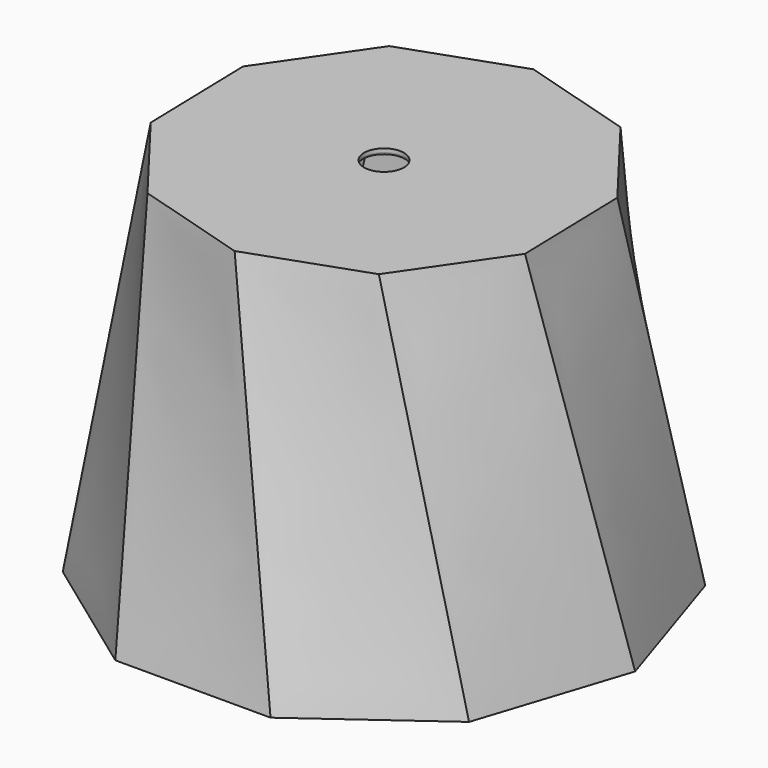
from build123d import *

# Parameters (mm, degrees)
F4_T     = -2.5
F5_R     = 8.1066370951
F6_DEPTH = 20
F7_R     = 1


with BuildPart() as f3:
    # F0 (on Top) → F3 section 0
    with BuildSketch(Plane.XY):
        Polygon((75.2863852023, -22.3556456815), (74.0482839108, 26.1661296438), (44.526254974, 64.6933327992), (-2.0032899712, 78.5098816708), (-47.7676462367, 62.3383241969), (-75.2863852023, 22.3556456815), (-74.0482839108, -26.1661296438), (-44.526254974, -64.6933327992), (2.0032899712, -78.5098816708), (47.7676462367, -62.3383241969), align=None)
    # F2 (on offset) → F3 section 1
    with BuildSketch(Plane.XY.offset(-150)):
        Polygon((31.5895679624, 97.2226932645), (-31.5895679624, 97.2226932645), (-82.7025626156, 60.0869289153), (-102.2259893063, 0), (-82.7025626156, -60.0869289153), (-31.5895679624, -97.2226932645), (31.5895679624, -97.2226932645), (82.7025626156, -60.0869289153), (102.2259893063, 0), (82.7025626156, 60.0869289153), align=None)
    loft()

    # F4
    f4_openings = [f3.faces().sort_by_distance(p)[0] for p in [
        (0, 0, -150),
    ]]
    offset(amount=F4_T, openings=f4_openings, kind=Kind.INTERSECTION)

    # F5 (on Top) → F6 (cut)
    with BuildSketch(Plane.XY):
        Circle(F5_R)
    extrude(amount=-F6_DEPTH, mode=Mode.SUBTRACT)

    # F7
    f7_edges = [f3.edges().sort_by_distance(p)[0] for p in [
        (-8.106637, 0, -2.5),
        (-57.297082, -44.392805, -2.5),
        (-20.260876, -69.592914, -2.5),
        (24.514295, -68.210894, -2.5),
        (59.925839, -40.774631, -2.5),
        (72.447749, 2.236154, -2.5),
        (57.297082, 44.392805, -2.5),
        (20.260876, 69.592914, -2.5),
        (-24.514295, 68.210894, -2.5),
        (-59.925839, 40.774631, -2.5),
        (-72.447749, -2.236154, -2.5),
    ]]
    fillet(f7_edges, radius=F7_R)


solid = f3.part
